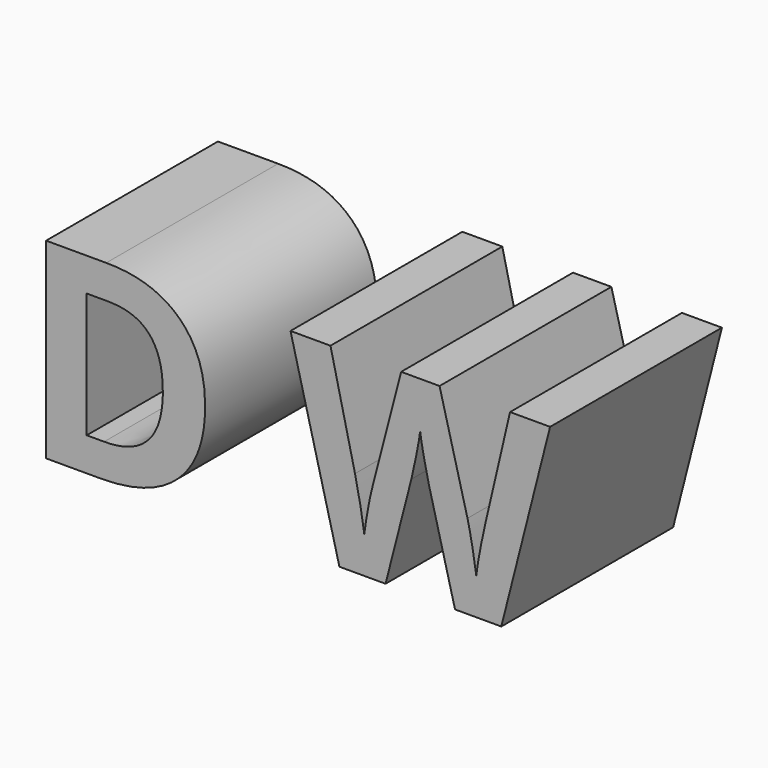
from build123d import *

# Parameters (mm, degrees)
F0_TEXT_SIZE = 31.75
F1_DEPTH     = 25.4


# Not quite as in the source:
# - Text() gives the source's letters only with a copy of the font that has no kerning and outlines rounded to 1/6400 em; it was checked with that copy


with BuildPart() as f1:
    # F0 (on Front) → F1 (new body)
    with BuildSketch(Plane.XZ):
        with Locations((-24.2454543401, 0)):
            Text('D W', F0_TEXT_SIZE, font='Open Sans', font_style=FontStyle.BOLD, text_align=(TextAlign.LEFT, TextAlign.BOTTOM))
    extrude(amount=F1_DEPTH)


solid = f1.part
